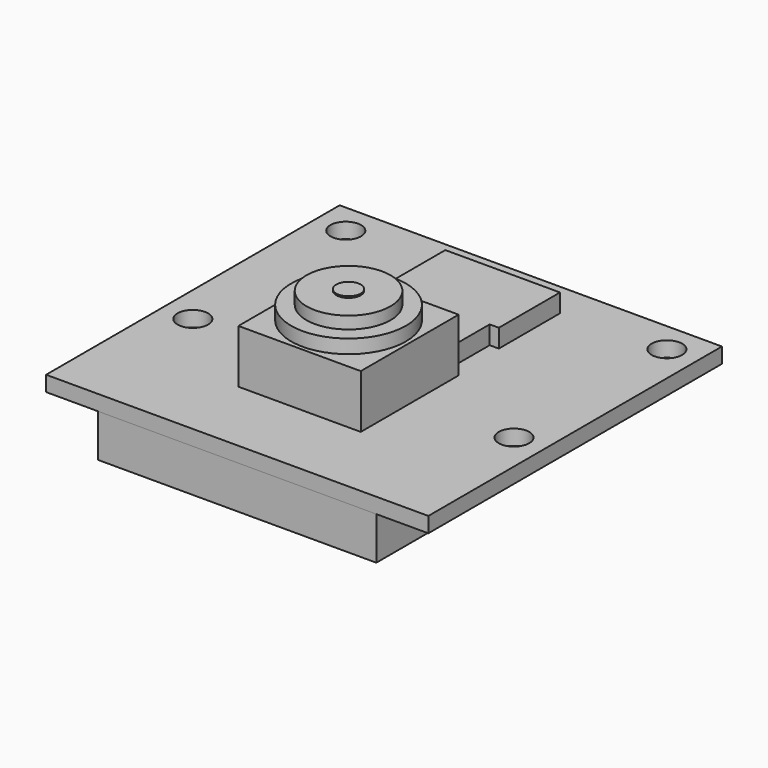
from build123d import *

# Parameters (mm, degrees)
F0_W      = 25
F0_H      = 24
F0_R      = 1
F1_DEPTH  = 1
F2_R      = 3.75
F2_R_2    = 2.75
F3_DEPTH  = 3.5
F4_DEPTH  = 4.4
F5_DEPTH  = 5.2
F6_R      = 0.8
F7_DEPTH  = 0.1
F8_W      = 18.2
F8_H      = 5.6
F9_DEPTH  = 2.8
F11_DEPTH = 1.2


with BuildPart() as f1:
    # F0 (on Top) → F1 (new body)
    with BuildSketch(Plane.XY):
        Rectangle(F0_W, F0_H)
        with Locations((-10.5, -2.5)):
            Circle(F0_R, mode=Mode.SUBTRACT)
        with Locations((10.5, -2.5)):
            Circle(F0_R, mode=Mode.SUBTRACT)
        with Locations((-10.5, 10)):
            Circle(F0_R, mode=Mode.SUBTRACT)
        with Locations((10.5, 10)):
            Circle(F0_R, mode=Mode.SUBTRACT)
    extrude(amount=F1_DEPTH)


with BuildPart() as f3:
    # F2 (on face) → F3 (new body)
    with BuildSketch(Plane.XY.offset(1)):
        Polygon((4, -6.9), (4, 1.1), (3.4, 1.1), (-3.4, 1.1), (-4, 1.1), (-4, -6.9), align=None)
        with Locations((0, -2.9)):
            Circle(F2_R, mode=Mode.SUBTRACT)
        with Locations((0, -2.9)):
            Circle(F2_R)
        with Locations((0, -2.9)):
            Circle(F2_R_2, mode=Mode.SUBTRACT)
        with Locations((0, -2.9)):
            Circle(F2_R_2)
    extrude(amount=F3_DEPTH)

    # F2 (on face) → F4 (join)
    with BuildSketch(Plane.XY.offset(1)):
        with Locations((0, -2.9)):
            Circle(F2_R)
        with Locations((0, -2.9)):
            Circle(F2_R_2, mode=Mode.SUBTRACT)
        with Locations((0, -2.9)):
            Circle(F2_R_2)
    extrude(amount=F4_DEPTH)

    # F2 (on face) → F5 (join)
    with BuildSketch(Plane.XY.offset(1)):
        with Locations((0, -2.9)):
            Circle(F2_R_2)
    extrude(amount=F5_DEPTH)


with BuildPart() as f7:
    # F6 (on face) → F7 (new body)
    with BuildSketch(Plane.XY.offset(6.2)):
        with Locations((0, -2.9)):
            Circle(F6_R)
    extrude(amount=F7_DEPTH)


with BuildPart() as f9:
    # F8 (on face) → F9 (new body)
    with BuildSketch(Plane(origin=(0, 0, 0), x_dir=(1, 0, 0), z_dir=(0, 0, -1))):
        with Locations((0, 9.2)):
            Rectangle(F8_W, F8_H)
    extrude(amount=F9_DEPTH)


with BuildPart() as f11:
    # F10 (on face) → F11 (new body)
    with BuildSketch(Plane.XY.offset(1)):
        Polygon((-3.15, 4.7), (-3.15, 1.1), (3.15, 1.1), (3.15, 4.7), (3.75, 4.7), (3.75, 9.7), (-3.75, 9.7), (-3.75, 4.7), align=None)
    extrude(amount=F11_DEPTH)


solid = Compound([f1.part, f3.part, f7.part, f9.part, f11.part])
